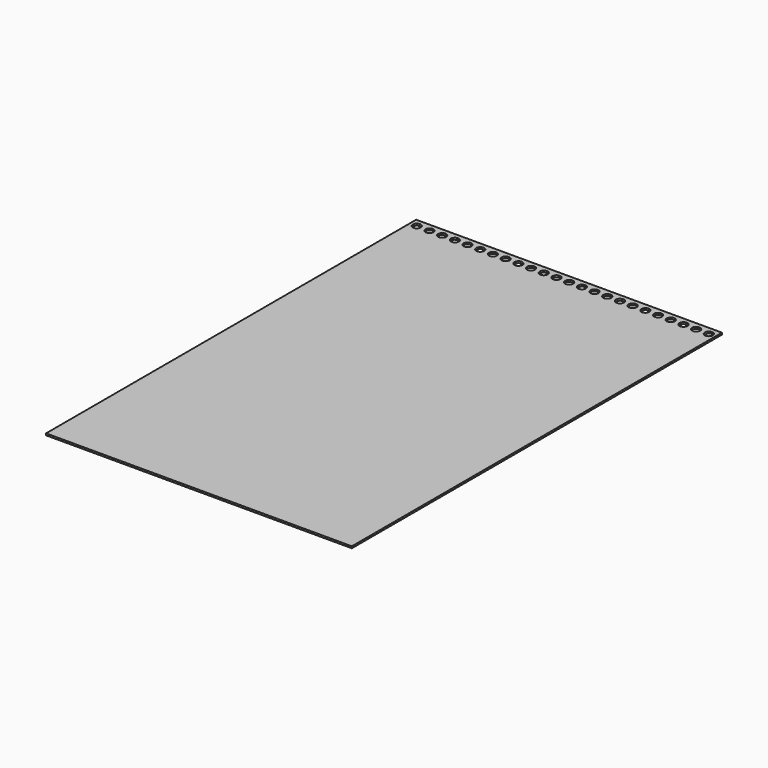
from build123d import *

# Parameters (mm, degrees)
F0_W     = 152.4
F0_H     = 230.6
F0_R     = 2
F1_DEPTH = 0.9


# Not quite as in the source:
# - a feature names something its author has since deleted; it is built from what else it names


with BuildPart() as f1:
    # F0 (on Top) → F1 (new body)
    with BuildSketch(Plane.XY):
        with Locations((76.2, 115.3)):
            Rectangle(F0_W, F0_H)
        with Locations((3.5, 226.6)):
            Circle(F0_R, mode=Mode.SUBTRACT)
        with Locations((9.83, 226.6)):
            Circle(F0_R, mode=Mode.SUBTRACT)
        with Locations((16.16, 226.6)):
            Circle(F0_R, mode=Mode.SUBTRACT)
        with Locations((22.49, 226.6)):
            Circle(F0_R, mode=Mode.SUBTRACT)
        with Locations((28.82, 226.6)):
            Circle(F0_R, mode=Mode.SUBTRACT)
        with Locations((35.15, 226.6)):
            Circle(F0_R, mode=Mode.SUBTRACT)
        with Locations((41.48, 226.6)):
            Circle(F0_R, mode=Mode.SUBTRACT)
        with Locations((47.81, 226.6)):
            Circle(F0_R, mode=Mode.SUBTRACT)
        with Locations((54.14, 226.6)):
            Circle(F0_R, mode=Mode.SUBTRACT)
        with Locations((60.47, 226.6)):
            Circle(F0_R, mode=Mode.SUBTRACT)
        with Locations((66.8, 226.6)):
            Circle(F0_R, mode=Mode.SUBTRACT)
        with Locations((73.13, 226.6)):
            Circle(F0_R, mode=Mode.SUBTRACT)
        with Locations((79.46, 226.6)):
            Circle(F0_R, mode=Mode.SUBTRACT)
        with Locations((85.79, 226.6)):
            Circle(F0_R, mode=Mode.SUBTRACT)
        with Locations((92.12, 226.6)):
            Circle(F0_R, mode=Mode.SUBTRACT)
        with Locations((98.45, 226.6)):
            Circle(F0_R, mode=Mode.SUBTRACT)
        with Locations((104.78, 226.6)):
            Circle(F0_R, mode=Mode.SUBTRACT)
        with Locations((111.11, 226.6)):
            Circle(F0_R, mode=Mode.SUBTRACT)
        with Locations((117.44, 226.6)):
            Circle(F0_R, mode=Mode.SUBTRACT)
        with Locations((123.77, 226.6)):
            Circle(F0_R, mode=Mode.SUBTRACT)
        with Locations((130.1, 226.6)):
            Circle(F0_R, mode=Mode.SUBTRACT)
        with Locations((136.43, 226.6)):
            Circle(F0_R, mode=Mode.SUBTRACT)
        with Locations((142.76, 226.6)):
            Circle(F0_R, mode=Mode.SUBTRACT)
        with Locations((149.09, 226.6)):
            Circle(F0_R, mode=Mode.SUBTRACT)
    extrude(amount=F1_DEPTH)


solid = f1.part
